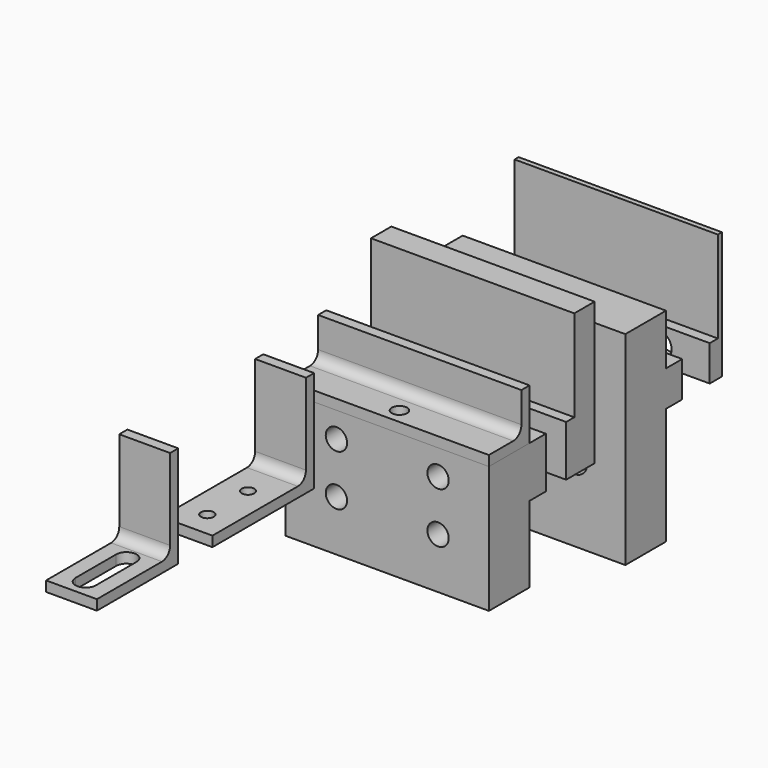
from build123d import *

# Parameters (mm, degrees)
F1_W      = 40
F1_H      = 40
F1_R      = 2.5
F2_DEPTH  = 10
F3_W      = 40
F3_H      = 7
F4_DEPTH  = 4
F5_R      = 2.5
F6_DEPTH  = 12
F8_DEPTH  = 40
F9_R      = 2.5
F10_DEPTH = 3
F12_DEPTH = 40
F14_DEPTH = 40
F18_DEPTH = 40
F15_R     = 2.1
F20_DEPTH = 10
F16_R     = 2.5
F21_DEPTH = 7
F19_R     = 1.25
F22_DEPTH = 12
F24_DEPTH = 10
F25_R     = 1.25
F26_DEPTH = 2
F28_DEPTH = 10
F30_DEPTH = 3
F31_R     = 2.1
F32_DEPTH = 14
F33_D     = 3


# Not quite as in the source:
# - a feature names something its author has since deleted; it is built from what else it names


with BuildPart() as f2:
    # F1 (on Front) → F2 (new body)
    with BuildSketch(Plane.XZ):
        with Locations((-20.3582742298, 3.9991794988)):
            Rectangle(F1_W, F1_H)
        with Locations((-30.3582742298, -1.0008205012)):
            Circle(F1_R, mode=Mode.SUBTRACT)
        with Locations((-10.3582742298, -1.0008205012)):
            Circle(F1_R, mode=Mode.SUBTRACT)
    extrude(amount=-F2_DEPTH)

    # F3 (on face) → F4 (join)
    with BuildSketch(Plane(origin=(0, 10, 0), x_dir=(-1, 0, 0), z_dir=(0, 1, 0))):
        with Locations((20.3582742298, 10.4991794988)):
            Rectangle(F3_W, F3_H)
    extrude(amount=F4_DEPTH)

    # F5 (on face) → F6 (cut)
    with BuildSketch(Plane(origin=(0, 14, 0), x_dir=(-1, 0, 0), z_dir=(0, 1, 0))):
        with Locations((10.3582742298, 10.4991794988)):
            Circle(F5_R)
        with Locations((30.3582742298, 10.4991794988)):
            Circle(F5_R)
    extrude(amount=-F6_DEPTH, mode=Mode.SUBTRACT)


with BuildPart() as f8:
    # F7 (on face) → F8 (new body)
    with BuildSketch(Plane(origin=(-40.3582742298, 0, 0), x_dir=(0, -1, 0), z_dir=(-1, 0, 0))):
        Polygon((-22.7574642788, 31.9991794988), (-23.7574642788, 31.9991794988), (-23.7574642788, 6.9991794988), (-20.7574642788, 6.9991794988), (-20.7574642788, 13.9991794988), (-22.7574642788, 13.9991794988), align=None)
    extrude(amount=-F8_DEPTH)

    # F9 (on face) → F10 (cut)
    with BuildSketch(Plane.XZ.offset(-20.7574642788)):
        with Locations((-30.3582742298, 10.4991794988)):
            Circle(F9_R)
        with Locations((-10.3582742298, 10.4991794988)):
            Circle(F9_R)
    extrude(amount=-F10_DEPTH, mode=Mode.SUBTRACT)


with BuildPart() as f12:
    # F11 (on offset) → F12 (new body)
    with BuildSketch(Plane.YZ.offset(-40)):
        Polygon((-20, 5), (-20, 15), (-34, 15), (-34, -10), (-24, -10), (-24, 5), align=None)
    extrude(amount=F12_DEPTH)

    # F15 (on face) → F20 (cut)
    with BuildSketch(Plane.XZ.offset(34)):
        with Locations((-30, 0)):
            Circle(F15_R)
        with Locations((-10, 0)):
            Circle(F15_R)
    extrude(amount=-F20_DEPTH, mode=Mode.SUBTRACT)


with BuildPart() as f14:
    # F13 (on offset) → F14 (new body)
    with BuildSketch(Plane.YZ.offset(-40)):
        Polygon((-8, 5), (-8, 33), (-13, 33), (-13, 15), (-15, 15), (-15, 5), align=None)
    extrude(amount=F14_DEPTH)

    # F16 (on face) → F21 (cut)
    with BuildSketch(Plane(origin=(0, -8, 0), x_dir=(-1, 0, 0), z_dir=(0, 1, 0))):
        with Locations((10, 10)):
            Circle(F16_R)
        with Locations((30, 10)):
            Circle(F16_R)
    extrude(amount=-F21_DEPTH, mode=Mode.SUBTRACT)


with BuildPart() as f18:
    # F17 (on offset) → F18 (new body)
    with BuildSketch(Plane.YZ.offset(-40)):
        with BuildLine():
            Line((-24, 15), (-24, 25))
            Line((-24, 25), (-26, 25))
            Line((-26, 25), (-26, 19))
            ThreePointArc((-26, 19), (-26.5857864376, 17.5857864376), (-28, 17))
            Line((-28, 17), (-34, 17))
            Line((-34, 17), (-34, 15))
            Line((-34, 15), (-24, 15))
        make_face()
    extrude(amount=F18_DEPTH)


with BuildPart() as f22_tool:
    # F19 (on face) → F22 (new body)
    with BuildSketch(Plane.XY.offset(17)):
        with Locations((-20, -31)):
            Circle(F19_R)
    extrude(amount=-F22_DEPTH)


with BuildPart() as f12_1:
    add(f12.part)

    # F22: cut by f22_tool
    add(f22_tool.part, mode=Mode.SUBTRACT)

    # F31 (on face) → F32 (cut)
    with BuildSketch(Plane(origin=(0, -20, 0), x_dir=(-1, 0, 0), z_dir=(0, 1, 0))):
        with Locations((30, 10)):
            Circle(F31_R)
        with Locations((10, 10)):
            Circle(F31_R)
    extrude(amount=-F32_DEPTH, mode=Mode.SUBTRACT)


with BuildPart() as f18_1:
    add(f18.part)

    # F22: cut by f22_tool
    add(f22_tool.part, mode=Mode.SUBTRACT)

    # F33 (through all)
    with Locations(Plane.XY.offset(17)):
        with Locations((-20, -31)):
            Hole(F33_D / 2)


with BuildPart() as f24:
    # F23 (on offset) → F24 (new body)
    with BuildSketch(Plane.YZ.offset(-40)):
        with BuildLine():
            Line((-39.4938005805, 3.6755907349), (-39.4938005805, 23.6755907349))
            Line((-39.4938005805, 23.6755907349), (-41.4938005805, 23.6755907349))
            Line((-41.4938005805, 23.6755907349), (-41.4938005805, 7.6755907349))
            ThreePointArc((-41.4938005805, 7.6755907349), (-42.0795870181, 6.2613771726), (-43.4938005805, 5.6755907349))
            Line((-43.4938005805, 5.6755907349), (-64.4938005805, 5.6755907349))
            Line((-64.4938005805, 5.6755907349), (-64.4938005805, 3.6755907349))
            Line((-64.4938005805, 3.6755907349), (-39.4938005805, 3.6755907349))
        make_face()
    extrude(amount=F24_DEPTH)

    # F25 (on face) → F26 (cut)
    with BuildSketch(Plane.XY.offset(5.6755907349)):
        with Locations((-35, -49.4938005805)):
            Circle(F25_R)
        with Locations((-35, -59.4938005805)):
            Circle(F25_R)
    extrude(amount=-F26_DEPTH, mode=Mode.SUBTRACT)


with BuildPart() as f28:
    # F27 (on offset) → F28 (new body)
    with BuildSketch(Plane.YZ.offset(-40)):
        with BuildLine():
            Line((-72.9045346379, 4.2176819406), (-72.9045346379, 24.2176819406))
            Line((-72.9045346379, 24.2176819406), (-74.9045346379, 24.2176819406))
            Line((-74.9045346379, 24.2176819406), (-74.9045346379, 8.2176819406))
            ThreePointArc((-74.9045346379, 8.2176819406), (-75.4903210756, 6.8034683783), (-76.9045346379, 6.2176819406))
            Line((-76.9045346379, 6.2176819406), (-92.9045346379, 6.2176819406))
            Line((-92.9045346379, 6.2176819406), (-92.9045346379, 4.2176819406))
            Line((-92.9045346379, 4.2176819406), (-72.9045346379, 4.2176819406))
        make_face()
    extrude(amount=F28_DEPTH)

    # F29 (on face) → F30 (cut)
    with BuildSketch(Plane.XY.offset(6.2176819406)):
        with BuildLine():
            Line((-37, -79.4045346379), (-37, -89.4045346379))
            ThreePointArc((-37, -89.4045346379), (-35, -91.4045346379), (-33, -89.4045346379))
            Line((-33, -89.4045346379), (-33, -79.4045346379))
            ThreePointArc((-33, -79.4045346379), (-35, -77.4045346379), (-37, -79.4045346379))
        make_face()
    extrude(amount=-F30_DEPTH, mode=Mode.SUBTRACT)


solid = Compound([f2.part, f8.part, f14.part, f12_1.part, f18_1.part, f24.part, f28.part])
